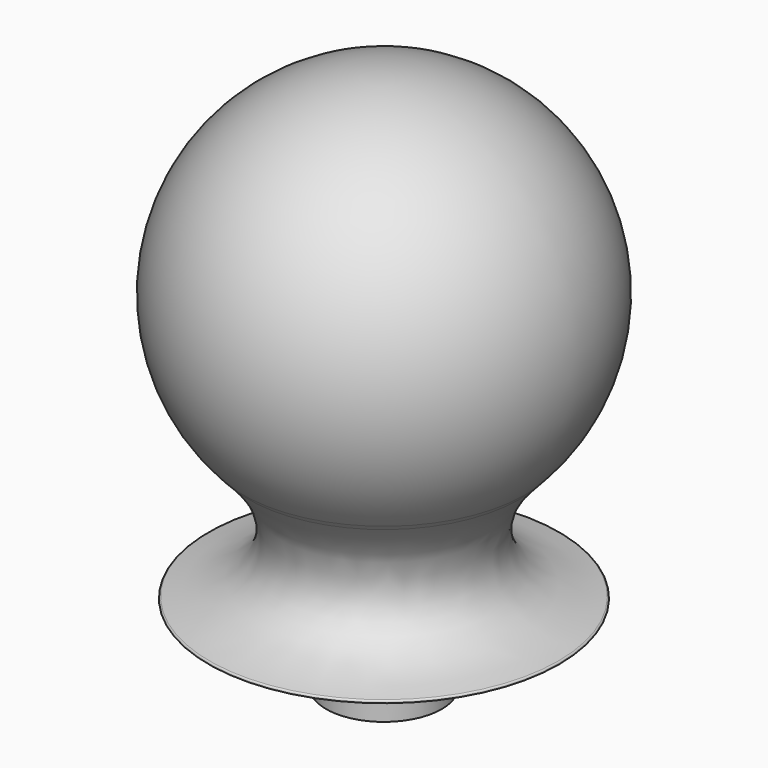
from build123d import *


# Not quite as in the source:
# - a fillet or chamfer that OpenCascade refuses, or shapes differently, is made with other operations: its cross-section is extruded or revolved along the edge and cut away or added


with BuildPart() as f1:
    # F0 (on Front) → F1 (revolve)
    with BuildSketch(Plane.XZ):
        with BuildLine():
            add(Edge.make_bspline(
                [(2.5003758306, 0.0177362721), (2.4404300279, -0.0413985663), (2.3744789771, -0.1082652449), (2.3049510778, -0.1817676763)],
                knots=[0, 0, 0, 0, 0.0510069156, 0.0510069156, 0.0510069156, 0.0510069156], degree=3))
            ThreePointArc((2.5003758306, 0.0177362721), (3.6940969816, 6.8849464932), (-2.1325040052, 10.7104225876))
            Line((-2.1325040052, 10.7104225876), (-2.132504005, -1.9895774124))
            ThreePointArc((-2.132504005, -1.9895774124), (0.2632831128, -1.5202835001), (2.3049510778, -0.1817676763))
        make_face()
        with BuildLine():
            ThreePointArc((2.3049510778, -0.1817676763), (2.4037603545, -0.0830901744), (2.5003758306, 0.0177362721))
            add(Edge.make_bspline(
                [(2.5003758306, 0.0177362721), (2.4404300279, -0.0413985663), (2.3744789771, -0.1082652449), (2.3049510778, -0.1817676763)],
                knots=[0, 0, 0, 0, 0.0510069156, 0.0510069156, 0.0510069156, 0.0510069156], degree=3))
        make_face()
        with BuildLine():
            add(Edge.make_bspline(
                [(2.3049510778, -0.1817676763), (1.9642470512, -0.5419479004), (1.0532611933, -1.6513807021), (1.0539929138, -3.8701076312), (3.2527025422, -4.5295774125), (5.0868722728, -4.5295774125)],
                knots=[0.0510069156, 0.0510069156, 0.0510069156, 0.0510069156, 0.300953508, 0.5847659526, 1, 1, 1, 1], degree=3))
            ThreePointArc((2.3049510778, -0.1817676763), (0.2632831128, -1.5202835001), (-2.132504005, -1.9895774124))
            Line((-2.132504005, -1.9895774124), (-2.1325040049, -4.5295774124))
            Line((-2.1325040049, -4.5295774124), (-0.2275040048, -4.5295774124))
            Line((-0.2275040048, -4.5295774124), (-0.1388052504, -4.5295774124))
            Line((-0.1388052504, -4.5295774124), (5.0868722728, -4.5295774125))
        make_face()
        Polygon((-0.2275040048, -4.5295774124), (-2.1325040049, -4.5295774124), (-2.1325040049, -7.0695774124), (-0.2275040049, -7.0695774124), (-0.1388052504, -4.5295774124), align=None)
    revolve(axis=Axis((-2.132504005, 0, 3.0904225876), (0, 0, -1)))

    # F2: fillet of radius 0.0508 on 1 edges, made by hand

    # F2_s1 → F2_t2 (revolve, cut)
    with BuildSketch(Plane.XZ):
        with BuildLine():
            ThreePointArc((3.6079651255, -4.4285482526), (3.651028038, -4.4825852127), (3.6003709491, -4.5295774123))
            Line((3.6003709491, -4.5295774123), (3.6003709491, -4.5305934123))
            Line((3.6003709491, -4.5305934123), (5.0868722728, -4.5305934125))
            Line((5.0868722728, -4.5305934125), (5.0868722728, -4.5285614125))
            ThreePointArc((5.0868722728, -4.5285614125), (4.3457025483, -4.5054914795), (3.6081170091, -4.4275436694))
            Line((3.6081170091, -4.4275436694), (3.6079651255, -4.4285482526))
        make_face()
    revolve(axis=Axis((-2.1325040049, 0, -4.5295774126), (0, 0, -1)), mode=Mode.SUBTRACT)


solid = f1.part
